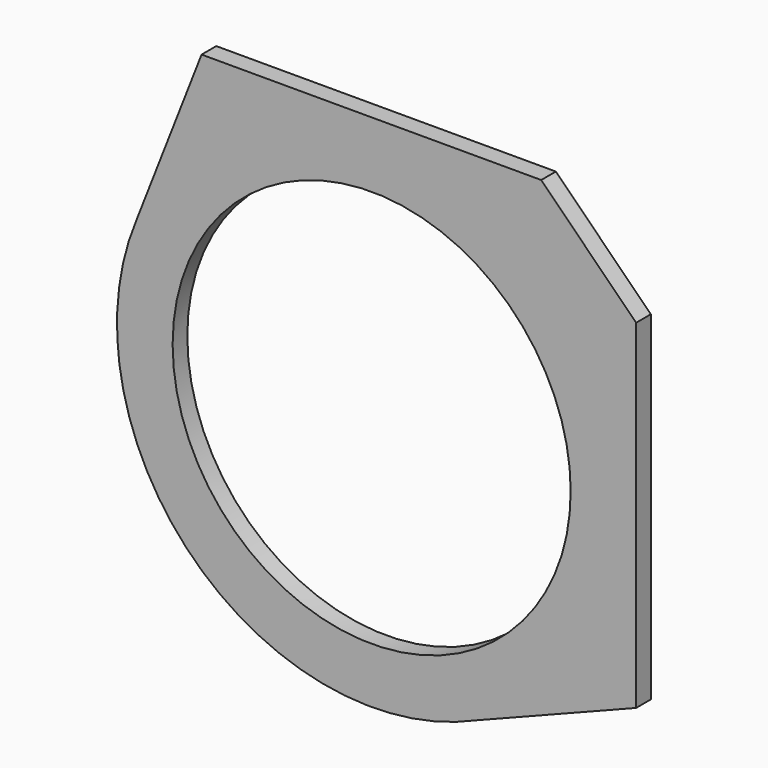
from build123d import *

# Parameters (mm, degrees)
F0_R     = 137.715625
F1_DEPTH = 12.7


# Not quite as in the source:
# - ends of sketch curves that miss each other by under 0.0002 mm in the source are joined


with BuildPart() as f1:
    # F0 (on Front) → F1 (new body)
    with BuildSketch(Plane.XZ):
        with BuildLine():
            Line((113.9265438, 179.606067), (-121.0729862, 179.606067))
            Line((-121.0729862, 179.606067), (-166.0250934, 64.4432544))
            ThreePointArc((-166.0250934, 64.4432544), (-131.6142451705, -124.2666526964), (54.7392664722, -169.7408508033))
            Line((54.7392664722, -169.7408508033), (179.606067, -120.6184532))
            Line((179.606067, -120.6184532), (179.606067, 114.0217684))
            Line((179.606067, 114.0217684), (113.9265438, 179.606067))
        make_face()
        with Locations((-3.393567, -3.393567)):
            Circle(F0_R, mode=Mode.SUBTRACT)
    extrude(amount=F1_DEPTH)


solid = f1.part
